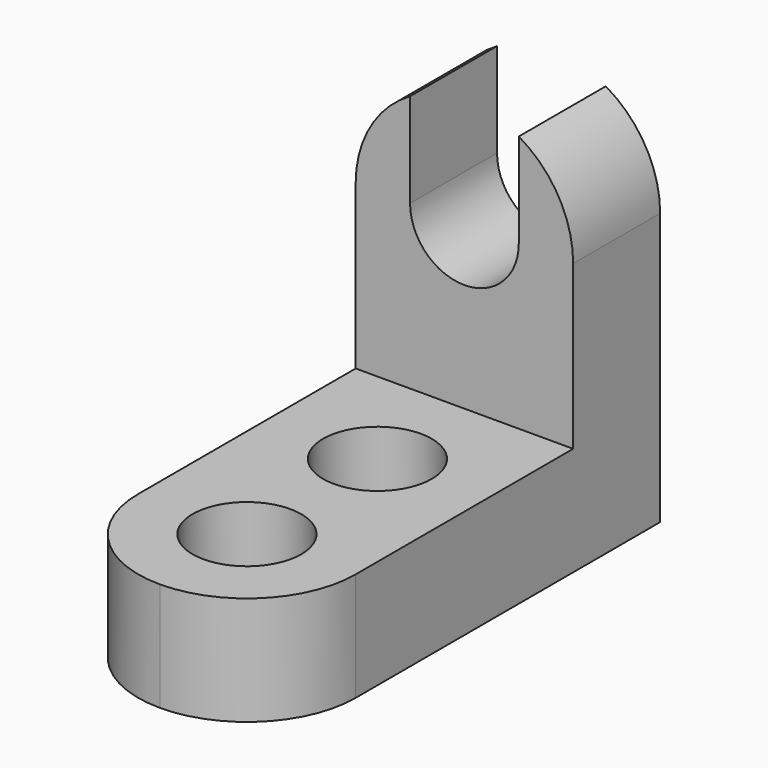
from build123d import *

# Parameters (mm, degrees)
F1_DEPTH    = 25.4
F2_T1_DEPTH = 76.2
F3_R        = 12.69999
F6_DEPTH    = 25.4
F4_R        = 6.35
F7_DEPTH    = 25.4


# Not quite as in the source:
# - a fillet or chamfer that OpenCascade refuses, or shapes differently, is made with other operations: its cross-section is extruded or revolved along the edge and cut away or added
# - a fillet or chamfer is up to 0.001 mm smaller than in the source, because OpenCascade refuses the exact size


with BuildPart() as f1:
    # F0 (on Right) → F1 (new body)
    with BuildSketch(Plane.YZ):
        Polygon((-57.15, 0), (0, 0), (0, 44.45), (-12.7, 44.45), (-12.7, 12.7), (-57.15, 12.7), align=None)
    extrude(amount=F1_DEPTH)

    # F2: fillet of radius 12.7 on 2 edges, made by hand

    # F2_s2 → F2_t1 (cut)
    with BuildSketch(Plane.XZ.offset(-31.75)):
        with BuildLine():
            ThreePointArc((12.7, 44.45), (3.7197438789, 40.7302561211), (0, 31.75))
            Line((0, 31.75), (0, 44.45))
            Line((0, 44.45), (12.7, 44.45))
        make_face()
        with BuildLine():
            ThreePointArc((12.7, 44.45), (21.6802561211, 40.7302561211), (25.4, 31.75))
            Line((25.4, 31.75), (25.4, 44.45))
            Line((25.4, 44.45), (12.7, 44.45))
        make_face()
    extrude(amount=F2_T1_DEPTH, mode=Mode.SUBTRACT)

    # F3 (radius 12.7 in the source; OpenCascade refuses exactly that, so slightly less here)
    f3_edges = [f1.edges().sort_by_distance(p)[0] for p in [
        (25.4, -57.15, 6.35),
        (0, -57.15, 6.35),
    ]]
    fillet(f3_edges, radius=F3_R)

    # F5 (on face) → F6 (cut)
    with BuildSketch(Plane(origin=(0, 0, 0), x_dir=(-1, 0, 0), z_dir=(0, 1, 0))):
        with BuildLine():
            ThreePointArc((-19.05, 31.75), (-12.7, 25.4), (-6.35, 31.75))
            ThreePointArc((-6.35, 31.75), (-12.7, 38.1), (-19.05, 31.75))
        make_face()
        with BuildLine():
            ThreePointArc((-19.05, 31.75), (-12.7, 38.1), (-6.35, 31.75))
            Line((-6.35, 31.75), (-6.35, 42.7485226281))
            ThreePointArc((-6.35, 42.7485226281), (-9.4129981272, 44.0172579939), (-12.7, 44.45))
            ThreePointArc((-12.7, 44.45), (-15.9870018728, 44.0172579939), (-19.05, 42.7485226281))
            Line((-19.05, 42.7485226281), (-19.05, 31.75))
        make_face()
    extrude(amount=-F6_DEPTH, mode=Mode.SUBTRACT)

    # F4 (on face) → F7 (cut)
    with BuildSketch(Plane.XY.offset(12.7)):
        with Locations((12.7, -44.45)):
            Circle(F4_R)
        with Locations((12.7, -25.4)):
            Circle(F4_R)
    extrude(amount=-F7_DEPTH, mode=Mode.SUBTRACT)


solid = f1.part
